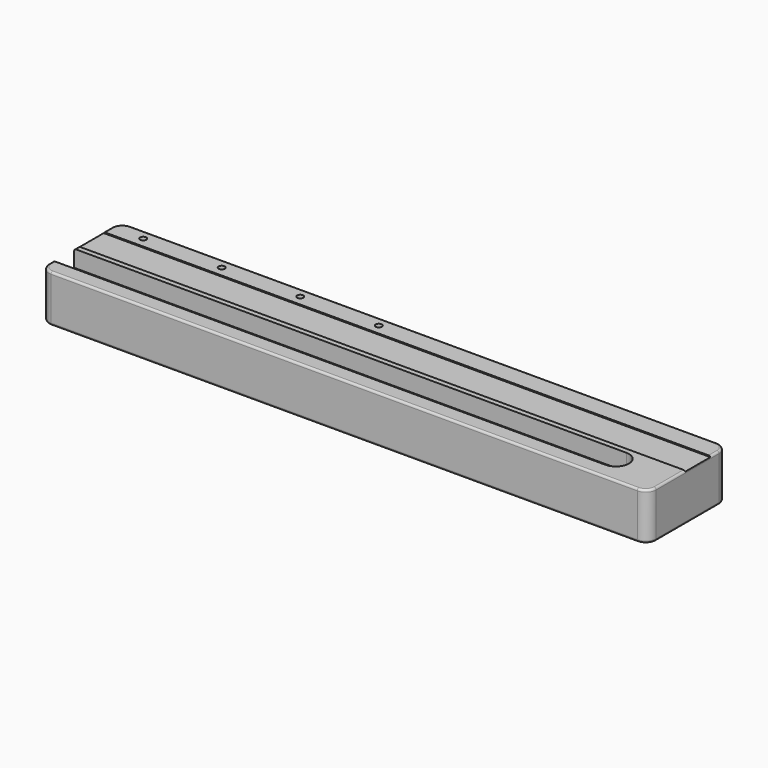
from build123d import *

# Parameters (mm, degrees)
F0_W      = 580
F0_H      = 95
F1_DEPTH  = 45
F3_START  = -40
F2_W      = 25
F2_H      = 16
F3_DEPTH  = 540.001
F6_D      = 6
F6_DEPTH  = 15
F6_TIP    = 1.8025818571
F7_R      = 10
F8_R      = 2
F9_R      = 12.49999
F5_W      = 30
F5_H      = 1
F10_DEPTH = 580.0010001


# Not quite as in the source:
# - a fillet or chamfer is up to 0.001 mm smaller than in the source, because OpenCascade refuses the exact size


with BuildPart() as f1:
    # F0 (on Top) → F1 (new body)
    with BuildSketch(Plane.XY):
        with Locations((43.9460686967, -446.140053056)):
            Rectangle(F0_W, F0_H)
    extrude(amount=F1_DEPTH)

    # F2 (on face) → F3 (cut)
    with BuildSketch(Plane.YZ.offset(333.9460686967).offset(F3_START)):
        with Locations((-466.140053056, 37)):
            Rectangle(F2_W, F2_H)
    extrude(amount=-F3_DEPTH, mode=Mode.SUBTRACT)

    # F6
    with Locations(Plane.XY.offset(45)):
        with Locations((-216.0539313033, -408.640053056), (-141.0539313033, -408.640053056), (-66.0539313033, -408.640053056), (8.9460686967, -408.640053056)):
            Hole(F6_D / 2, depth=F6_DEPTH)
            with Locations((0, 0, -(F6_DEPTH + F6_TIP / 2))):  # 118° drill point
                Cone(0, F6_D / 2, F6_TIP, mode=Mode.SUBTRACT)

    # F7
    f7_edges = [f1.edges().sort_by_distance(p)[0] for p in [
        (-246.053931, -493.640053, 22.5),
        (333.946069, -493.640053, 22.5),
        (333.946069, -398.640053, 22.5),
        (-246.053931, -398.640053, 22.5),
    ]]
    fillet(f7_edges, radius=F7_R)

    # F8
    f8_edges = [f1.edges().sort_by_distance(p)[0] for p in [
        (43.946069, -398.640053, 45),
        (43.946069, -493.640053, 45),
        (43.946069, -493.640053, 0),
    ]]
    fillet(f8_edges, radius=F8_R)

    # F9 (radius 12.5 in the source; OpenCascade refuses exactly that, so slightly less here)
    f9_edges = [f1.edges().sort_by_distance(p)[0] for p in [
        (293.946069, -453.640053, 37),
        (293.946069, -478.640053, 37),
    ]]
    fillet(f9_edges, radius=F9_R)

    # F5 (on face) → F10 (cut, through all)
    with BuildSketch(Plane.YZ.offset(333.9460686967)):
        with Locations((-433.640053056, 44.5)):
            Rectangle(F5_W, F5_H)
    extrude(amount=-F10_DEPTH, mode=Mode.SUBTRACT)


solid = f1.part
